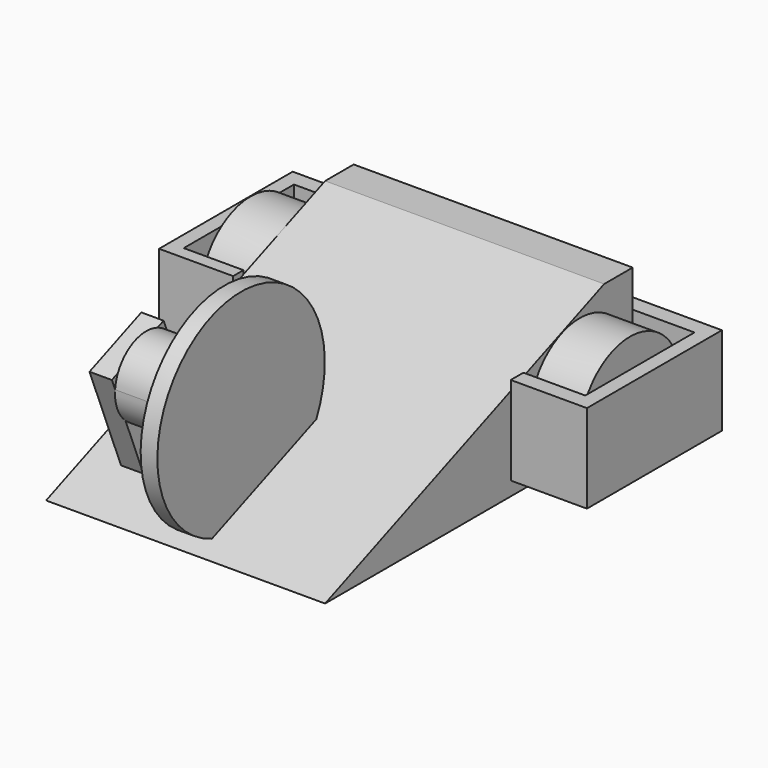
from build123d import *

# Parameters (mm, degrees)
F1_DEPTH  = 1270
F3_DEPTH  = 457.2
F5_DEPTH  = 457.2
F7_DEPTH  = 693.42
F8_W      = 130.3792857361
F8_H      = 805.9367705113
F9_DEPTH  = 1391.92
F10_W     = 148.9687260818
F10_H     = 805.9367705113
F11_DEPTH = 3776.98
F12_W     = 130.5909924316
F12_H     = 805.9367705113
F13_DEPTH = 1371.6
F14_W     = 117.6594177246
F14_H     = 805.9367705113
F15_DEPTH = 543.56
F16_W     = 203.2
F16_H     = 635
F17_DEPTH = 965.2
F19_DEPTH = 711.2
F20_R     = 952.5
F21_DEPTH = 152.4
F22_DEPTH = 325.12


with BuildPart() as f1:
    # F0 (on Right) → F1 (new body, symmetric)
    with BuildSketch(Plane.YZ):
        Polygon((3175, 1270), (0, 0), (3175, 0), align=None)
    extrude(amount=F1_DEPTH, both=True)

    # F2 (on face) → F3 (join)
    with BuildSketch(Plane.YZ.offset(1270)):
        with BuildLine():
            ThreePointArc((3175, 38.5786582061), (3390.6275667745, 248.389447831), (3469.8190059662, 538.6385321617))
            ThreePointArc((3469.8190059662, 538.6385321617), (3390.6275667745, 828.8876164925), (3175, 1038.6984061173))
            Line((3175, 1038.6984061173), (3175, 38.5786582061))
        make_face()
        with BuildLine():
            Line((3175, 38.5786582061), (3175, 1038.6984061173))
            ThreePointArc((3175, 1038.6984061173), (2377.2058441792, 773.2729768036), (2707.3195775098, 0))
            Line((2707.3195775098, 0), (3089.3184344226, 0))
            ThreePointArc((3089.3184344226, 0), (3132.9534506081, 17.5253703748), (3175, 38.5786582061))
        make_face()
        with BuildLine():
            Line((3089.3184344226, 0), (2707.3195775098, 0))
            ThreePointArc((2707.3195775098, 0), (2898.3190059662, -32.8614678383), (3089.3184344226, 0))
        make_face()
    extrude(amount=F3_DEPTH)

    # F4 (on face) → F5 (join)
    with BuildSketch(Plane(origin=(-1270, 0, 0), x_dir=(0, -1, 0), z_dir=(-1, 0, 0))):
        with BuildLine():
            Line((-3175, 38.5786582061), (-3175, 1038.6984061173))
            ThreePointArc((-3175, 1038.6984061173), (-3469.8190059662, 538.6385321617), (-3175, 38.5786582061))
        make_face()
        with BuildLine():
            ThreePointArc((-3089.3184344226, 0), (-2898.3190059662, -32.8614678383), (-2707.3195775098, 0))
            Line((-2707.3195775098, 0), (-3089.3184344226, 0))
        make_face()
        with BuildLine():
            ThreePointArc((-2707.3195775098, 0), (-2431.538316904, 208.8991831016), (-2326.8190059662, 538.6385321617))
            ThreePointArc((-2326.8190059662, 538.6385321617), (-2608.0699216354, 1030.94709297), (-3175, 1038.6984061173))
            Line((-3175, 1038.6984061173), (-3175, 38.5786582061))
            ThreePointArc((-3175, 38.5786582061), (-3132.9534506081, 17.5253703748), (-3089.3184344226, 0))
            Line((-3089.3184344226, 0), (-2707.3195775098, 0))
        make_face()
    extrude(amount=F5_DEPTH)

    # F6 (on face) → F7 (join)
    with BuildSketch(Plane.YZ.offset(1270)):
        Polygon((2112.5289201736, 127), (2256.6655874252, 127), (2256.6655874252, 902.6662349701), (2112.5289201736, 845.0115680695), align=None)
        Polygon((2112.5289201736, 845.0115680695), (2256.6655874252, 902.6662349701), (2256.6655874252, 932.9367705113), (2112.5289201736, 932.9367705113), align=None)
    extrude(amount=F7_DEPTH)

    # F8 (on face) → F9 (join)
    with BuildSketch(Plane(origin=(0, 2256.6655874252, 0), x_dir=(-1, 0, 0), z_dir=(0, 1, 0))):
        with Locations((-1898.230357132, 529.9683852557)):
            Rectangle(F8_W, F8_H)
    extrude(amount=F9_DEPTH)

    # F10 (on face) → F11 (join)
    with BuildSketch(Plane(origin=(1833.0407142639, 0, 0), x_dir=(0, -1, 0), z_dir=(-1, 0, 0))):
        with Locations((-3574.1012243843, 529.9683852557)):
            Rectangle(F10_W, F10_H)
    extrude(amount=F11_DEPTH)

    # F12 (on face) → F13 (join)
    with BuildSketch(Plane.XZ.offset(-3499.6168613434)):
        with Locations((-1878.6437895203, 529.9683852557)):
            Rectangle(F12_W, F12_H)
    extrude(amount=F13_DEPTH)

    # F14 (on face) → F15 (join)
    with BuildSketch(Plane.YZ.offset(-1813.3482933044)):
        with Locations((2186.8465702057, 529.9683852557)):
            Rectangle(F14_W, F14_H)
    extrude(amount=F15_DEPTH)

    # F16 (on face) → F17 (join)
    with BuildSketch(Plane(origin=(0, 0, 0), x_dir=(1, 0, 0), z_dir=(0, -0.3713906764, 0.9284766909))):
        with Locations((-863.6, 825.5)):
            Rectangle(F16_W, F16_H)
    extrude(amount=F17_DEPTH)

    # F18 (on face) → F19 (join)
    with BuildSketch(Plane.YZ.offset(-762)):
        with BuildLine():
            ThreePointArc((858.6660271031, 930.9566195196), (859.6662288573, 946.3274518263), (859.9998380943, 961.7271789091))
            ThreePointArc((859.9998380943, 961.7271789091), (828.5370859157, 1107.9680917029), (739.7163477975, 1228.3308177835))
            Line((739.7163477975, 1228.3308177835), (858.6660271031, 930.9566195196))
        make_face()
        with BuildLine():
            Line((858.6660271031, 930.9566195196), (739.7163477975, 1228.3308177835))
            ThreePointArc((739.7163477975, 1228.3308177835), (689.5258400202, 1265.3383173921), (633.6423229739, 1293.0091435588))
            Line((633.6423229739, 1293.0091435588), (182.3401320437, 1112.4882671867))
            ThreePointArc((182.3401320437, 1112.4882671867), (160.9560860217, 1053.9104157926), (150.1336490854, 992.4977382986))
            Line((150.1336490854, 992.4977382986), (269.083328391, 695.1235400347))
            ThreePointArc((269.083328391, 695.1235400347), (636.4663626058, 631.5608676303), (858.6660271031, 930.9566195196))
        make_face()
        with BuildLine():
            Line((182.3401320437, 1112.4882671867), (633.6423229739, 1293.0091435588))
            ThreePointArc((633.6423229739, 1293.0091435588), (372.3333135827, 1291.8934901879), (182.3401320437, 1112.4882671867))
        make_face()
        with BuildLine():
            ThreePointArc((150.1336490854, 992.4977382986), (174.2335268155, 829.6606543976), (269.083328391, 695.1235400347))
            Line((269.083328391, 695.1235400347), (150.1336490854, 992.4977382986))
        make_face()
    extrude(amount=F19_DEPTH)

    # F20 (on face) → F21 (join)
    with BuildSketch(Plane.YZ.offset(-50.8)):
        with Locations((504.3998380943, 961.7271789091)):
            Circle(F20_R)
    extrude(amount=F21_DEPTH)

    # F22 (add): a face of the model
    f22_faces = [f1.faces().sort_by_distance(p)[0] for p in [
        (0, 3175, 635),
    ]]
    extrude(f22_faces, amount=F22_DEPTH)


solid = f1.part
